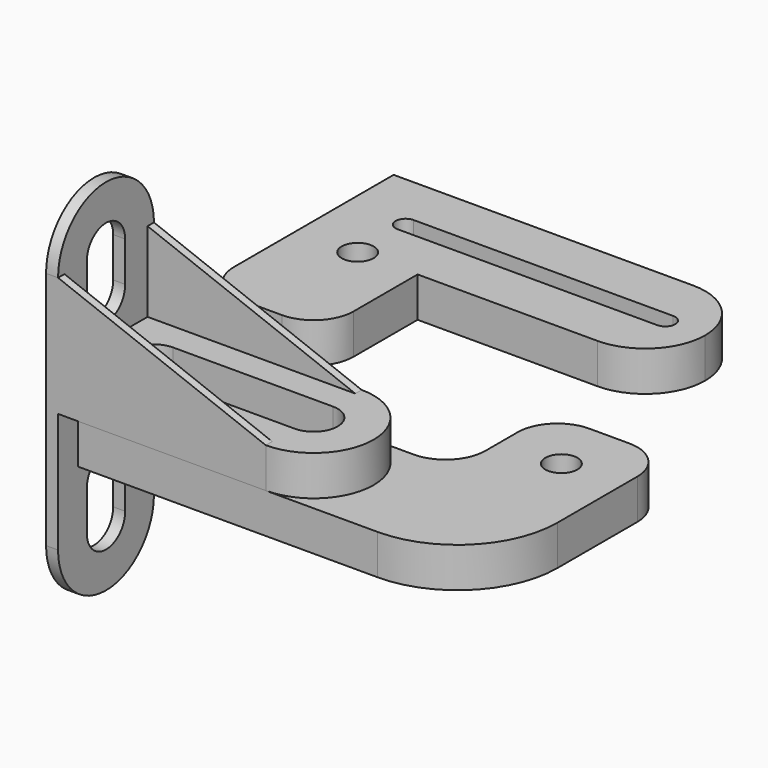
from build123d import *

# Parameters (mm, degrees)
F1_DEPTH  = 10
F3_DEPTH  = 3
F4_R      = 4
F5_DEPTH  = 10
F6_R      = 25
F7_R      = 10
F8_DEPTH  = 30
F9_W      = 23.3748118877
F9_H      = 20
F10_DEPTH = 30
F13_R     = 4
F14_DEPTH = 10
F15_R     = 14.99999
F16_R     = 10


# Not quite as in the source:
# - a fillet or chamfer is up to 0.001 mm smaller than in the source, because OpenCascade refuses the exact size


with BuildPart() as f1:
    # F0 (on Top) → F1 (new body)
    with BuildSketch(Plane.XY):
        with BuildLine():
            Line((52, 15), (0, 15))
            Line((0, 15), (0, 13))
            Line((0, 13), (52, 13))
            ThreePointArc((52, 13), (65, 0), (52, -13))
            Line((52, -13), (0, -13))
            Line((0, -13), (0, -15))
            Line((0, -15), (52, -15))
            ThreePointArc((52, -15), (67, 0), (52, 15))
        make_face()
        with BuildLine():
            Line((52, 13), (0, 13))
            Line((0, 13), (0, -13))
            Line((0, -13), (52, -13))
            ThreePointArc((52, -13), (65, 0), (52, 13))
        make_face()
        with BuildLine():
            Line((12, 6), (52, 6))
            ThreePointArc((52, 6), (58, 0), (52, -6))
            Line((52, -6), (12, -6))
            ThreePointArc((12, -6), (6, 0), (12, 6))
        make_face(mode=Mode.SUBTRACT)
    extrude(amount=F1_DEPTH)

    # F2 (on Right) → F3 (join)
    with BuildSketch(Plane.YZ):
        with BuildLine():
            Line((-15, 30), (-15, 0))
            Line((-15, 0), (-15, -30))
            ThreePointArc((-15, -30), (0, -45), (15, -30))
            Line((15, -30), (15, 0))
            Line((15, 0), (15, 30))
            ThreePointArc((15, 30), (0, 45), (-15, 30))
        make_face()
        with BuildLine():
            Line((6, -20), (6, -30))
            ThreePointArc((6, -30), (0, -36), (-6, -30))
            Line((-6, -30), (-6, -20))
            ThreePointArc((-6, -20), (0, -14), (6, -20))
        make_face(mode=Mode.SUBTRACT)
        with BuildLine():
            Line((-6, 20), (-6, 30))
            ThreePointArc((-6, 30), (0, 36), (6, 30))
            Line((6, 30), (6, 20))
            ThreePointArc((6, 20), (0, 14), (-6, 20))
        make_face(mode=Mode.SUBTRACT)
    extrude(amount=-F3_DEPTH)

    # F0 (on Top) → F8 (join)
    with BuildSketch(Plane.XY):
        with BuildLine():
            Line((52, 15), (0, 15))
            Line((0, 15), (0, 13))
            Line((0, 13), (52, 13))
            ThreePointArc((52, 13), (65, 0), (52, -13))
            Line((52, -13), (0, -13))
            Line((0, -13), (0, -15))
            Line((0, -15), (52, -15))
            ThreePointArc((52, -15), (67, 0), (52, 15))
        make_face()
    extrude(amount=F8_DEPTH)

    # F9 (on face) → F10 (cut)
    with BuildSketch(Plane.XZ.offset(15)):
        with Locations((63.6874059439, 20)):
            Rectangle(F9_W, F9_H)
        Polygon((52, 30), (0, 30), (52, 10), align=None)
    extrude(amount=-F10_DEPTH, mode=Mode.SUBTRACT)


with BuildPart() as f5:
    # F4 (on face) → F5 (new body)
    with BuildSketch(Plane(origin=(0, 0, 0), x_dir=(1, 0, 0), z_dir=(0, 0, -1))):
        with BuildLine():
            Line((52, 15), (5, 15))
            Line((5, 15), (5, -15))
            Line((5, -15), (52, -15))
            ThreePointArc((52, -15), (67, 0), (52, 15))
        make_face()
        with BuildLine():
            Line((52, -6), (12, -6))
            ThreePointArc((12, -6), (6, 0), (12, 6))
            Line((12, 6), (52, 6))
            ThreePointArc((52, 6), (58, 0), (52, -6))
        make_face(mode=Mode.SUBTRACT)
        with BuildLine():
            Line((105, 15), (52, 15))
            ThreePointArc((52, 15), (67, 0), (52, -15))
            Line((52, -15), (75, -15))
            Line((75, -15), (75, -45))
            Line((75, -45), (105, -45))
            Line((105, -45), (105, 15))
        make_face()
        with Locations((90, -30)):
            Circle(F4_R, mode=Mode.SUBTRACT)
        with BuildLine():
            ThreePointArc((12, 6), (6, 0), (12, -6))
            Line((12, -6), (52, -6))
            ThreePointArc((52, -6), (58, 0), (52, 6))
            Line((52, 6), (12, 6))
        make_face()
        with Locations((20, 0)):
            Circle(F4_R, mode=Mode.SUBTRACT)
    extrude(amount=F5_DEPTH)

    # F6
    f6_edges = [f5.edges().sort_by_distance(p)[0] for p in [
        (105, -15, -5),
    ]]
    fillet(f6_edges, radius=F6_R)

    # F7
    f7_edges = [f5.edges().sort_by_distance(p)[0] for p in [
        (75, 45, -5),
        (105, 45, -5),
        (75, 15, -5),
    ]]
    fillet(f7_edges, radius=F7_R)


with BuildPart() as f14:
    # F13 (on Top) → F14 (new body)
    with BuildSketch(Plane.XY):
        Polygon((90, 90), (0, 90), (0, 30), (30, 30), (30, 60), (90, 60), align=None)
        with Locations((15, 60)):
            Circle(F13_R, mode=Mode.SUBTRACT)
        with BuildLine():
            Line((15, 77.5), (80, 77.5))
            ThreePointArc((80, 77.5), (82.5, 75), (80, 72.5))
            Line((80, 72.5), (15, 72.5))
            ThreePointArc((15, 72.5), (12.5, 75), (15, 77.5))
        make_face(mode=Mode.SUBTRACT)
    extrude(amount=F14_DEPTH)

    # F15 (radius 15 in the source; OpenCascade refuses exactly that, so slightly less here)
    f15_edges = [f14.edges().sort_by_distance(p)[0] for p in [
        (90, 60, 5),
        (90, 90, 5),
    ]]
    fillet(f15_edges, radius=F15_R)

    # F16
    f16_edges = [f14.edges().sort_by_distance(p)[0] for p in [
        (0, 30, 5),
        (30, 30, 5),
    ]]
    fillet(f16_edges, radius=F16_R)


solid = Compound([f1.part, f5.part, f14.part])
